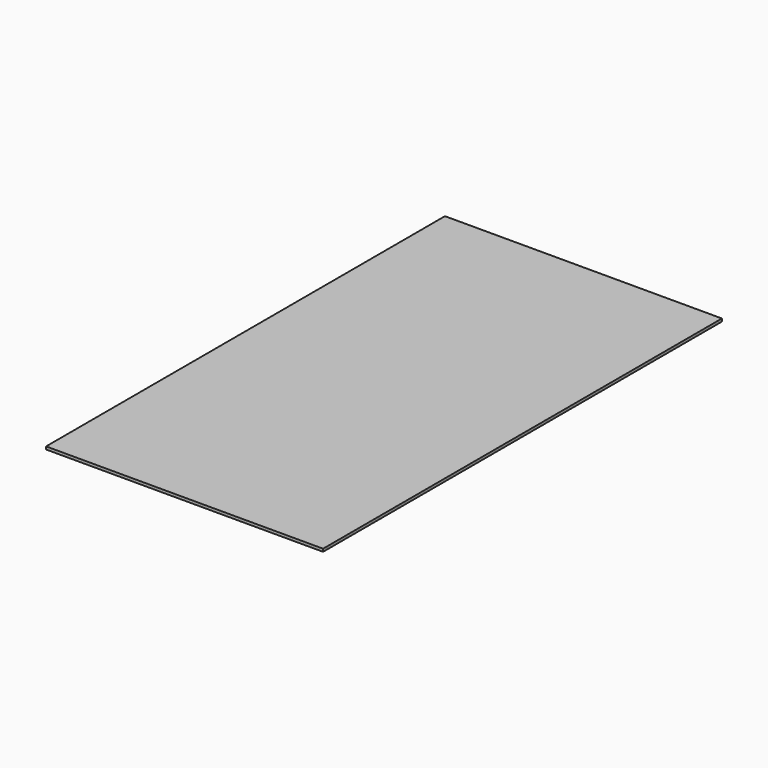
from build123d import *

# Parameters (mm, degrees)
F0_W     = 10000
F0_H     = 18000
F1_DEPTH = 100


# Not quite as in the source:
# - a feature names something its author has since deleted; it is built from what else it names


with BuildPart() as f1:
    # F0 (on Top) → F1 (new body)
    with BuildSketch(Plane.XY):
        with Locations((0, -5000)):
            Rectangle(F0_W, F0_H)
    extrude(amount=-F1_DEPTH)


solid = f1.part
